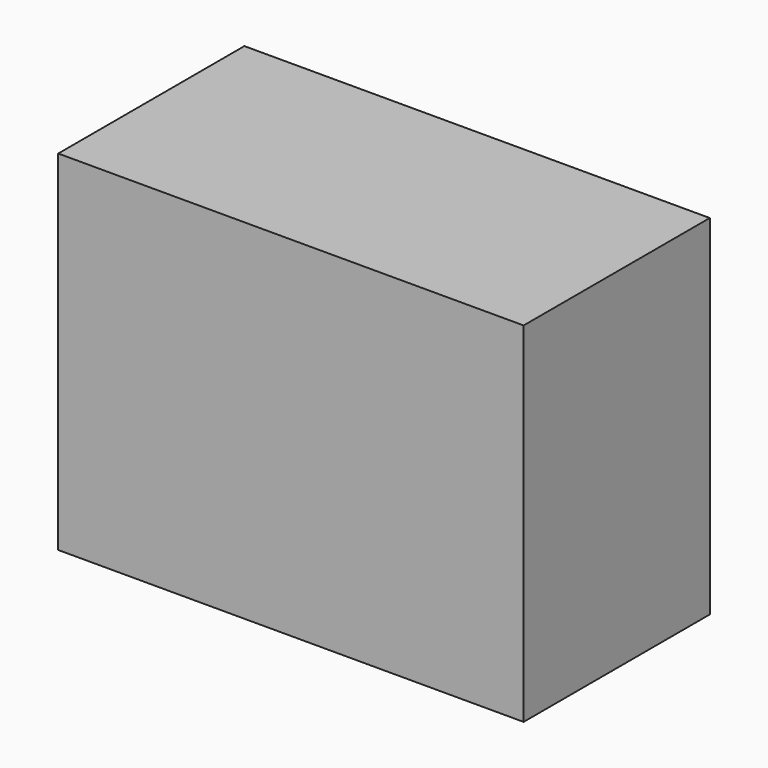
from build123d import *

# Parameters (mm, degrees)
F1_W     = 101.6
F1_H     = 76.2
F2_DEPTH = 50.8


# Not quite as in the source:
# - a feature names something its author has since deleted; it is built from what else it names


with BuildPart() as f2:
    # F1 (on Front) → F2 (new body)
    with BuildSketch(Plane.XZ):
        Rectangle(F1_W, F1_H)
    extrude(amount=F2_DEPTH)


solid = f2.part
